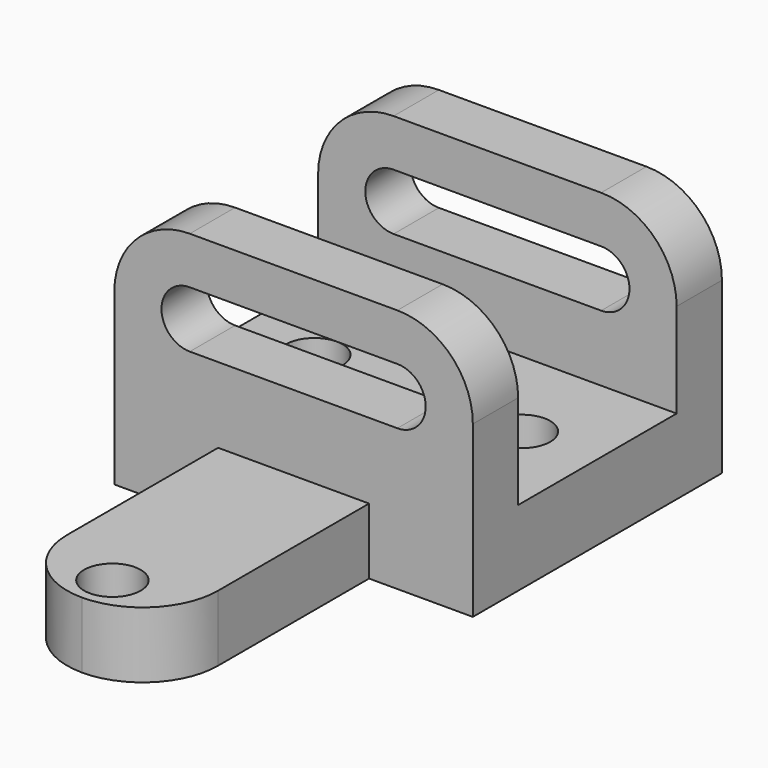
from build123d import *

# Parameters (mm, degrees)
F1_DEPTH  = 76
F2_R      = 16
F4_DEPTH  = 66.001
F5_R      = 6
F6_DEPTH  = 16.001
F8_W      = 32
F8_H      = 14
F9_DEPTH  = 56
F11_R     = 15.99999
F10_R     = 6
F12_DEPTH = 14.001


# Not quite as in the source:
# - a fillet or chamfer is up to 0.001 mm smaller than in the source, because OpenCascade refuses the exact size


with BuildPart() as f1:
    # F0 (on Right) → F1 (new body)
    with BuildSketch(Plane.YZ):
        Polygon((-33.8781030774, 28.9183304161), (-33.8781030774, -23.0816695839), (32.1218969226, -23.0816695839), (32.1218969226, 28.9183304161), (20.1218969226, 28.9183304161), (20.1218969226, -7.0816695839), (-21.8781030774, -7.0816695839), (-21.8781030774, 28.9183304161), align=None)
    extrude(amount=F1_DEPTH)

    # F2
    f2_edges = [f1.edges().sort_by_distance(p)[0] for p in [
        (76, -27.878103, 28.91833),
        (76, 26.121897, 28.91833),
        (0, 26.121897, 28.91833),
        (0, -27.878103, 28.91833),
    ]]
    fillet(f2_edges, radius=F2_R)

    # F3 (on face) → F4 (cut, through all)
    with BuildSketch(Plane.XZ.offset(33.8781030774)):
        with BuildLine():
            Line((60, 18.9183304161), (16, 18.9183304161))
            ThreePointArc((16, 18.9183304161), (10, 12.9183304161), (16, 6.9183304161))
            Line((16, 6.9183304161), (60, 6.9183304161))
            ThreePointArc((60, 6.9183304161), (66, 12.9183304161), (60, 18.9183304161))
        make_face()
    extrude(amount=-F4_DEPTH, mode=Mode.SUBTRACT)

    # F5 (on face) → F6 (cut, through all)
    with BuildSketch(Plane.XY.offset(-7.0816695839)):
        with Locations((60, -0.8781030774)):
            Circle(F5_R)
        with Locations((16, -0.8781030774)):
            Circle(F5_R)
    extrude(amount=-F6_DEPTH, mode=Mode.SUBTRACT)


with BuildPart() as f9:
    # F8 (on offset) → F9 (new body)
    with BuildSketch(Plane.XZ.offset(89.8781030774)):
        with Locations((38, -16.0816695839)):
            Rectangle(F8_W, F8_H)
    extrude(amount=-F9_DEPTH)

    # F11 (radius 16 in the source; OpenCascade refuses exactly that, so slightly less here)
    f11_edges = [f9.edges().sort_by_distance(p)[0] for p in [
        (54, -89.878103, -16.08167),
        (22, -89.878103, -16.08167),
    ]]
    fillet(f11_edges, radius=F11_R)

    # F10 (on face) → F12 (cut, through all)
    with BuildSketch(Plane.XY.offset(-9.0816695839)):
        with Locations((38, -81.8781030774)):
            Circle(F10_R)
    extrude(amount=-F12_DEPTH, mode=Mode.SUBTRACT)


solid = Compound([f1.part, f9.part])
